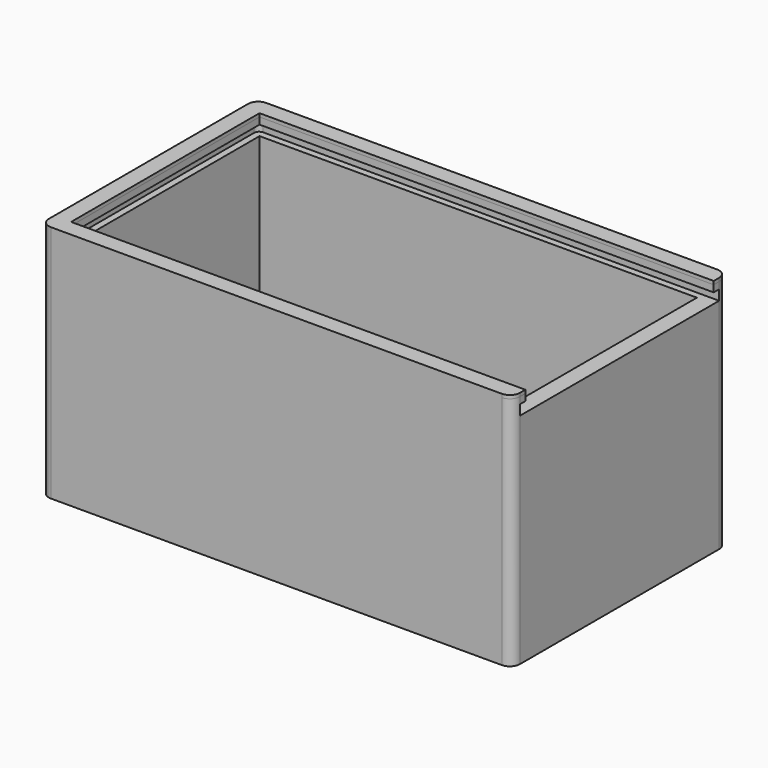
from build123d import *

# Parameters (mm, degrees)
F0_W      = 140
F0_H      = 80
F0_W_2    = 130
F0_H_2    = 70
F1_DEPTH  = 70
F2_DEPTH  = 5
F3_W      = 5
F3_H      = 70
F4_DEPTH  = 5
F6_DEPTH  = 2
F8_DEPTH  = 2
F10_DEPTH = 2
F11_R     = 2.99999
F12_R     = 1.5
F13_DEPTH = 1


# Not quite as in the source:
# - a fillet or chamfer is up to 0.001 mm smaller than in the source, because OpenCascade refuses the exact size


with BuildPart() as f1:
    # F0 (on Top) → F1 (new body)
    with BuildSketch(Plane.XY):
        Rectangle(F0_W, F0_H)
        Rectangle(F0_W_2, F0_H_2, mode=Mode.SUBTRACT)
    extrude(amount=F1_DEPTH)

    # F0 (on Top) → F2 (join)
    with BuildSketch(Plane.XY):
        Rectangle(F0_W_2, F0_H_2)
    extrude(amount=F2_DEPTH)

    # F3 (on face) → F4 (cut)
    with BuildSketch(Plane.XY.offset(70)):
        with Locations((67.5, 0)):
            Rectangle(F3_W, F3_H)
    extrude(amount=-F4_DEPTH, mode=Mode.SUBTRACT)

    # F5 (on face) → F6 (cut)
    with BuildSketch(Plane.XZ.offset(-35)):
        Polygon((65, 65), (70, 65), (70, 68), (-65, 68), (-65, 65), align=None)
    extrude(amount=-F6_DEPTH, mode=Mode.SUBTRACT)

    # F7 (on face) → F8 (cut)
    with BuildSketch(Plane.YZ.offset(-65)):
        Polygon((35, 65), (37, 65), (37, 68), (35, 68), (-35, 68), (-35, 65), align=None)
    extrude(amount=-F8_DEPTH, mode=Mode.SUBTRACT)

    # F9 (on face) → F10 (cut)
    with BuildSketch(Plane(origin=(0, -35, 0), x_dir=(-1, 0, 0), z_dir=(0, 1, 0))):
        Polygon((65, 65), (67, 65), (67, 68), (65, 68), (-70, 68), (-70, 65), (-65, 65), align=None)
    extrude(amount=-F10_DEPTH, mode=Mode.SUBTRACT)

    # F11 (radius 3 in the source; OpenCascade refuses exactly that, so slightly less here)
    f11_edges = [f1.edges().sort_by_distance(p)[0] for p in [
        (-70, -40, 35),
        (-70, 40, 35),
        (70, 40, 35),
        (70, -40, 35),
    ]]
    fillet(f11_edges, radius=F11_R)

    # F12
    f12_edges = [f1.edges().sort_by_distance(p)[0] for p in [
        (-67, -37, 66.5),
        (-67, 37, 66.5),
    ]]
    fillet(f12_edges, radius=F12_R)

    # F13 (add): a face of the model
    f13_faces = [f1.faces().sort_by_distance(p)[0] for p in [
        (-68.3875484503, 0, 70),
    ]]
    extrude(f13_faces, amount=F13_DEPTH)


solid = f1.part
